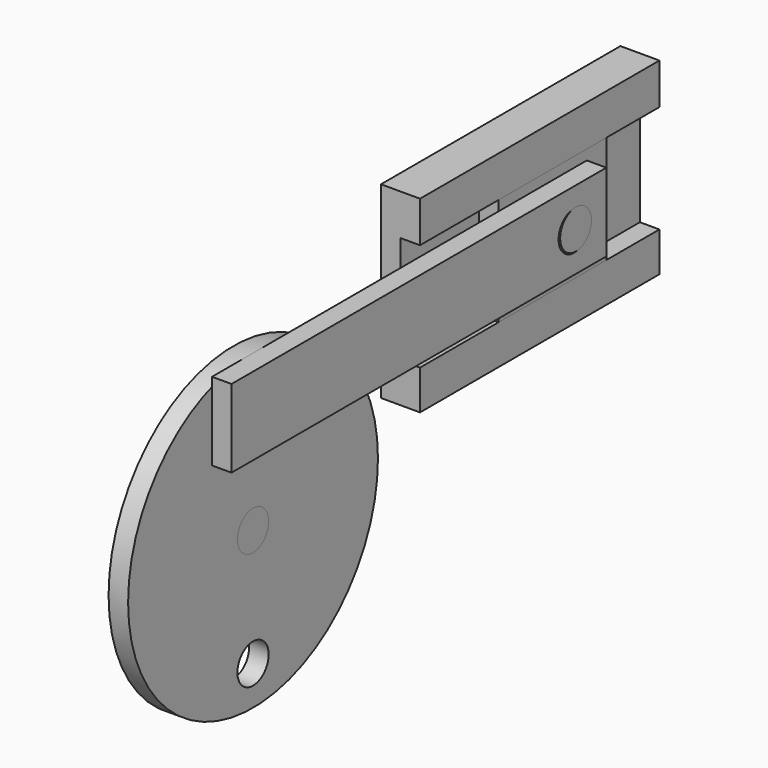
from build123d import *

# Parameters (mm, degrees)
F0_R          = 25.4
F0_R_2        = 3.175
F1_DEPTH      = 3.175
F2_R          = 3.175
F3_DEPTH      = 3.175
F4_W          = 76.2
F4_H          = 12.7
F4_R          = 3.175
F5_DEPTH      = 3.175
F6_R          = 3.175
F7_DEPTH      = 3.175
F7_DEPTH_BACK = 3.175
F8_W          = 21.9192807563
F8_H          = 17.51816459
F8_R          = 3.175
F9_DEPTH      = 3.175
F10_R         = 3.175
F11_DEPTH     = 6.35
F13_W         = 48.6749447882
F13_H         = 6.6694635898
F13_H_2       = 17.51816459
F13_H_3       = 6.4215252642
F14_DEPTH     = 3.175
F15_DEPTH     = 3.175


with BuildPart() as f1:
    # F0 (on Right) → F1 (new body)
    with BuildSketch(Plane.YZ):
        with Locations((-67.8579392607, 0)):
            Circle(F0_R)
        with Locations((-67.8579392607, 0)):
            Circle(F0_R_2, mode=Mode.SUBTRACT)
        with Locations((-67.8579392607, -19.0500002354)):
            Circle(F0_R_2, mode=Mode.SUBTRACT)
        with Locations((-67.8579392607, 19.0500002354)):
            Circle(F0_R_2, mode=Mode.SUBTRACT)
    extrude(amount=F1_DEPTH)


with BuildPart() as f3:
    # F2 (on face) → F3 (new body)
    with BuildSketch(Plane.YZ.offset(3.175)):
        with Locations((-67.8579392607, 0)):
            Circle(F2_R)
    extrude(amount=-F3_DEPTH)


with BuildPart() as f5:
    # F4 (on face) → F5 (new body)
    with BuildSketch(Plane.YZ.offset(3.175)):
        with Locations((-38.1, 19.05)):
            Rectangle(F4_W, F4_H)
        with Locations((-67.8579392607, 19.0500002354)):
            Circle(F4_R, mode=Mode.SUBTRACT)
        with Locations((-6.5324339084, 19.05)):
            Circle(F4_R, mode=Mode.SUBTRACT)
    extrude(amount=F5_DEPTH)

    # F6 (on face) → F7 (join, two sides)
    with BuildSketch(Plane(origin=(3.175, 0, 0), x_dir=(0, -1, 0), z_dir=(-1, 0, 0))) as f7_sk:
        with Locations((67.8579392607, 19.0500002354)):
            Circle(F6_R)
    extrude(amount=F7_DEPTH)
    extrude(f7_sk.sketch, amount=-F7_DEPTH_BACK)


with BuildPart() as f9:
    # F8 (on Right) → F9 (new body)
    with BuildSketch(Plane.YZ):
        with Locations((-6.9793609437, 18.2802686468)):
            Rectangle(F8_W, F8_H)
        with Locations((-6.2026930973, 19.1000849009)):
            Circle(F8_R, mode=Mode.SUBTRACT)
    extrude(amount=F9_DEPTH)

    # F10 (on face) → F11 (join)
    with BuildSketch(Plane(origin=(0, 0, 0), x_dir=(0, -1, 0), z_dir=(-1, 0, 0))):
        with Locations((6.2026930973, 19.1000849009)):
            Circle(F10_R)
    extrude(amount=-F11_DEPTH)

    # F12: union 


with BuildPart() as f14:
    # F13 (on face) → F14 (new body)
    with BuildSketch(Plane(origin=(0, 0, 0), x_dir=(0, -1, 0), z_dir=(-1, 0, 0))):
        with Locations((9.5699708909, 30.3740827367)):
            Rectangle(F13_W, F13_H)
        with Locations((9.5699708909, 18.2802686468)):
            Rectangle(F13_W, F13_H_2)
        with Locations((9.5699708909, 6.3104237197)):
            Rectangle(F13_W, F13_H_3)
    extrude(amount=F14_DEPTH)

    # F13 (on face) → F15 (join)
    with BuildSketch(Plane(origin=(0, 0, 0), x_dir=(0, -1, 0), z_dir=(-1, 0, 0))):
        Polygon((33.907443285, 33.7088145316), (-14.7675015032, 33.7088145316), (-14.7675015032, 27.0393509418), (-3.9802794345, 27.0393509418), (17.9390013218, 27.0393509418), (33.907443285, 27.0393509418), align=None)
        Polygon((-3.9802794345, 9.5211863518), (-14.7675015032, 9.5211863518), (-14.7675015032, 3.0996610876), (33.907443285, 3.0996610876), (33.907443285, 9.5211863518), (17.9390013218, 9.5211863518), align=None)
    extrude(amount=-F15_DEPTH)


solid = Compound([f1.part, f3.part, f5.part, f9.part, f14.part])
